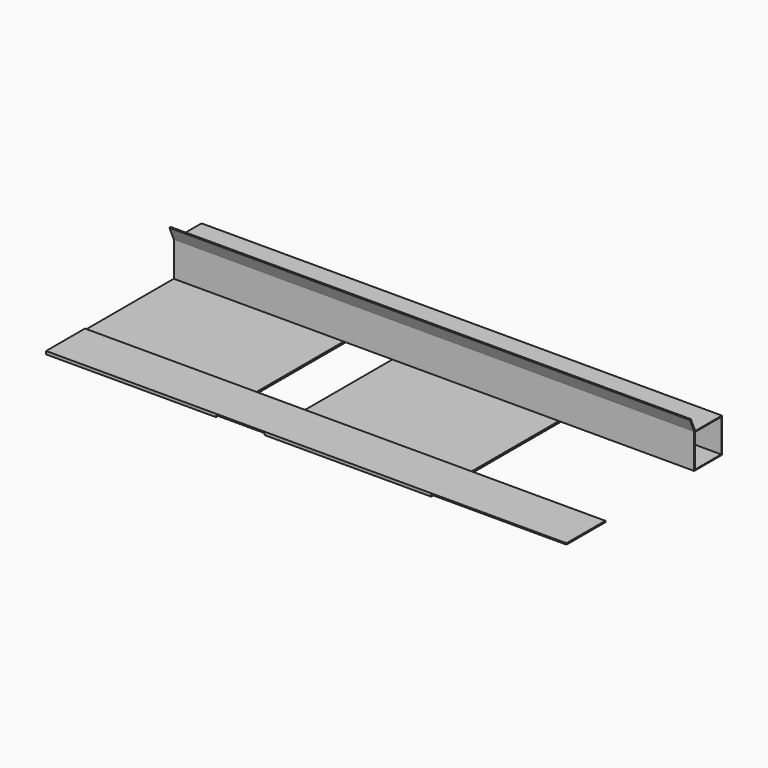
from build123d import *

# Parameters (mm, degrees)
F0_W     = 127
F0_H     = 127
F0_W_2   = 120.904
F0_H_2   = 120.904
F1_DEPTH = 1905
F3_DEPTH = 1905
F4_W     = 622.3
F4_H     = 6.35
F4_W_2   = 609.6
F5_DEPTH = 711.2
F6_W     = 1282.7
F6_H     = 177.8
F6_W_2   = 622.3
F7_DEPTH = 4.7625


with BuildPart() as f1:
    # F0 (on Right) → F1 (new body)
    with BuildSketch(Plane.YZ):
        with Locations((4.929526709, 15.0205540939)):
            Rectangle(F0_W, F0_H)
        with Locations((4.929526709, 15.0205540939)):
            Rectangle(F0_W_2, F0_H_2, mode=Mode.SUBTRACT)
    extrude(amount=F1_DEPTH)

    # F2 (on face) → F3 (join)
    with BuildSketch(Plane.YZ.offset(1905)):
        Polygon((-78.5117968917, 123.9730939269), (-58.570473291, 78.5205540939), (-53.4608645662, 78.5205540939), (-73.8704177914, 125.0403363069), align=None)
    extrude(amount=-F3_DEPTH)

    # F4 (on face) → F5 (join)
    with BuildSketch(Plane(origin=(0, 68.429526709, 0), x_dir=(-1, 0, 0), z_dir=(0, 1, 0))):
        with Locations((-311.15, -51.6544459061)):
            Rectangle(F4_W, F4_H)
        with Locations((-1104.9, -51.6544459061)):
            Rectangle(F4_W_2, F4_H)
    extrude(amount=-F5_DEPTH)

    # F6 (on face) → F7 (join)
    with BuildSketch(Plane.XY.offset(-48.4794459061)):
        with Locations((1263.65, -553.870473291)):
            Rectangle(F6_W, F6_H)
        with Locations((311.15, -553.870473291)):
            Rectangle(F6_W_2, F6_H)
    extrude(amount=F7_DEPTH)


solid = f1.part
